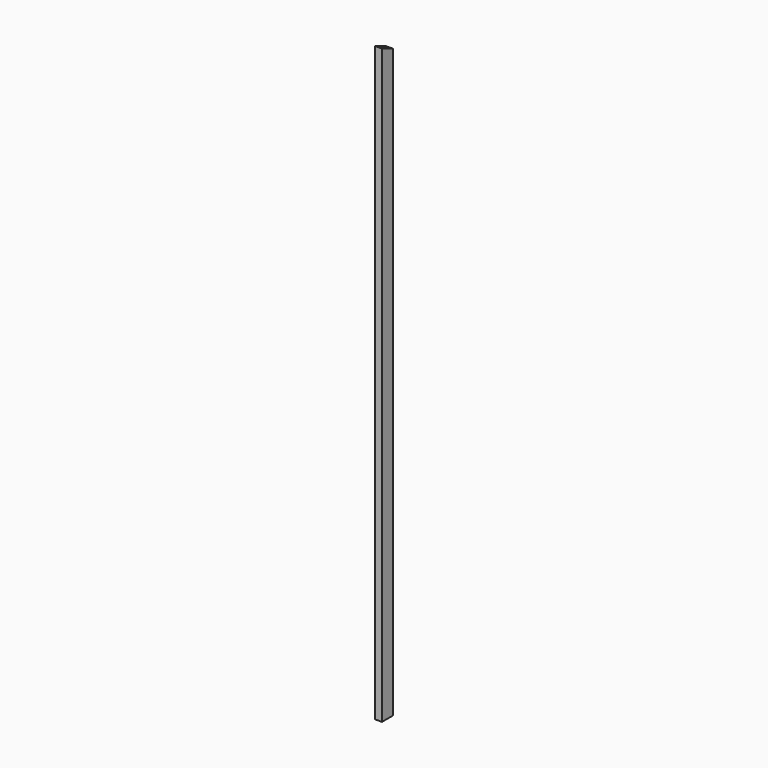
from build123d import *

# Parameters (mm, degrees)
F0_W        = 50
F0_H        = 100
F0_W_2      = 44
F0_H_2      = 94
F1_DEPTH    = 4362
F2_T1_DEPTH = 568.5605442995


# Not quite as in the source:
# - a fillet or chamfer that OpenCascade refuses, or shapes differently, is made with other operations: its cross-section is extruded or revolved along the edge and cut away or added


with BuildPart() as f1:
    # F0 (on Top) → F1 (new body)
    with BuildSketch(Plane.XY):
        Rectangle(F0_W, F0_H)
        Rectangle(F0_W_2, F0_H_2, mode=Mode.SUBTRACT)
    extrude(amount=F1_DEPTH)

    # F2: chamfer of 100 x 41 on 1 edges, made by hand

    # F2_s2 → F2_t1 (cut)
    with BuildSketch(Plane.YZ.offset(-284.2802721497)):
        Polygon((50, 4321), (-50, 4362), (50, 4362), align=None)
    extrude(amount=F2_T1_DEPTH, mode=Mode.SUBTRACT)


solid = f1.part
